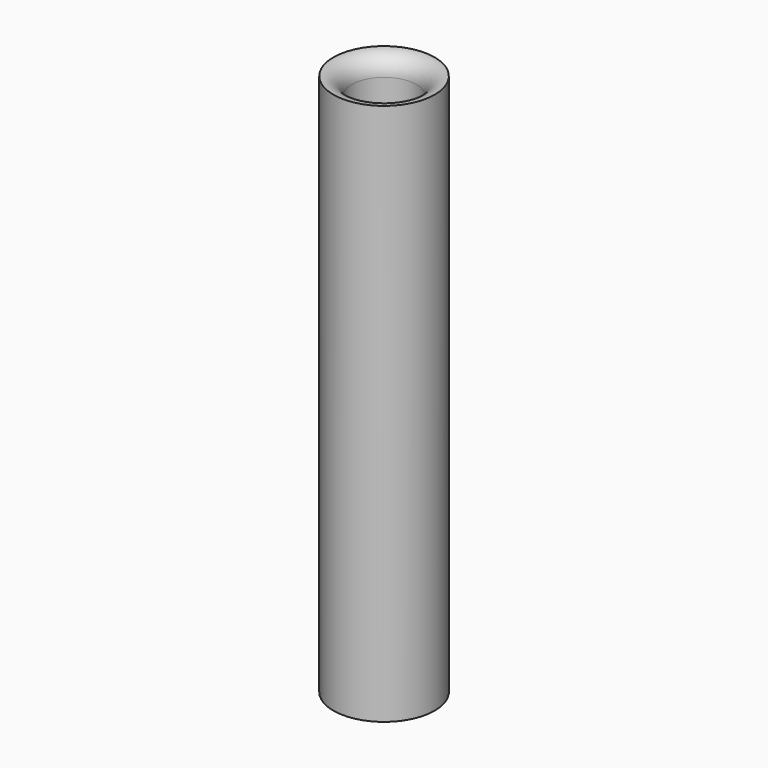
from build123d import *

# Parameters (mm, degrees)
F0_R     = 14
F0_R_2   = 9
F1_DEPTH = 150
F2_R     = 4.99999


# Not quite as in the source:
# - a fillet or chamfer is up to 0.001 mm smaller than in the source, because OpenCascade refuses the exact size


with BuildPart() as f1:
    # F0 (on Top) → F1 (new body)
    with BuildSketch(Plane.XY):
        Circle(F0_R)
        Circle(F0_R_2, mode=Mode.SUBTRACT)
    extrude(amount=F1_DEPTH)

    # F2 (radius 5 in the source; OpenCascade refuses exactly that, so slightly less here)
    f2_edges = [f1.edges().sort_by_distance(p)[0] for p in [
        (-9, 0, 150),
        (-9, 0, 0),
    ]]
    fillet(f2_edges, radius=F2_R)


solid = f1.part
